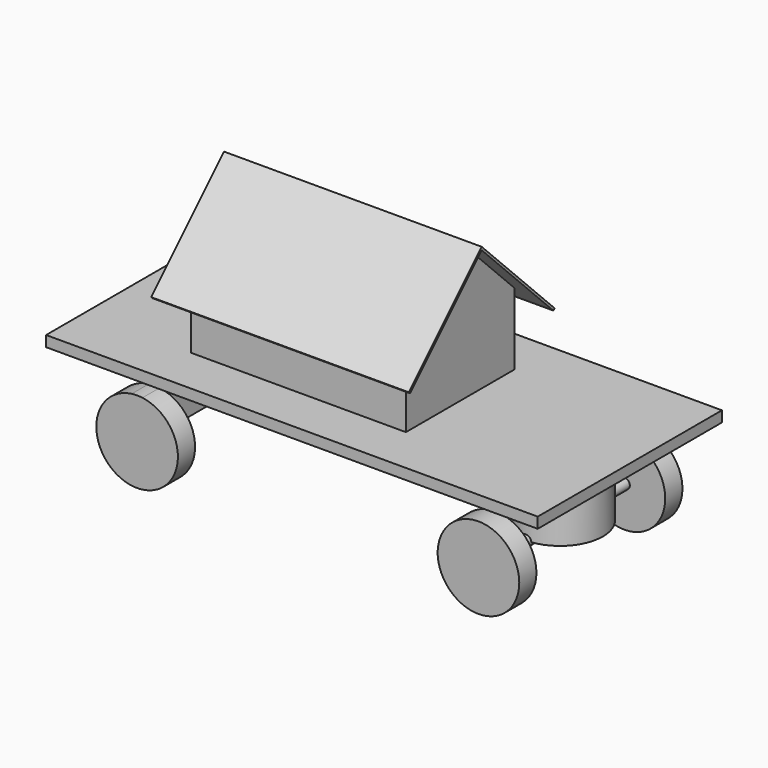
from build123d import *

# Parameters (mm, degrees)
F0_W      = 4580
F0_H      = 2145
F1_DEPTH  = 100
F2_W      = 100
F2_H      = 580
F3_DEPTH  = 450
F4_DEPTH  = 750
F6_DEPTH  = 200
F8_DEPTH  = 200
F9_R      = 400
F10_DEPTH = 580
F11_R     = 50
F12_DEPTH = 750
F13_R     = 380
F13_R_2   = 50
F14_DEPTH = 200
F15_R     = 380
F15_R_2   = 50
F16_DEPTH = 200
F17_W     = 2000
F17_H     = 1265
F18_DEPTH = 2000
F20_DEPTH = 2000
F22_DEPTH = 2200
F23_DEPTH = 200


# Not quite as in the source:
# - a feature names something its author has since deleted; it is built from what else it names


with BuildPart() as f1:
    # F0 (on Top) → F1 (new body)
    with BuildSketch(Plane.XY):
        Rectangle(F0_W, F0_H)
    extrude(amount=F1_DEPTH)

    # F2 (on Front) → F3 (join, symmetric)
    with BuildSketch(Plane.XZ):
        with Locations((-1540, -290)):
            Rectangle(F2_W, F2_H)
    extrude(amount=F3_DEPTH, both=True)

    # F2 (on Front) → F4 (join, symmetric)
    with BuildSketch(Plane.XZ):
        with Locations((-1540, -290)):
            Rectangle(F2_W, F2_H)
    extrude(amount=F4_DEPTH, both=True)

    # F5 (on face) → F6 (join)
    with BuildSketch(Plane.XZ.offset(750)):
        with BuildLine():
            ThreePointArc((-1590, -204.43457899), (-1790.399680511, -866.9628615859), (-1160, -581.1307430267))
            ThreePointArc((-1160, -581.1307430267), (-1254.1678814409, -330.7310625158), (-1490, -204.43457899))
            Line((-1490, -204.43457899), (-1490, -580))
            Line((-1490, -580), (-1590, -580))
            Line((-1590, -580), (-1590, -204.43457899))
        make_face()
        with BuildLine():
            Line((-1490, -580), (-1490, -204.43457899))
            ThreePointArc((-1490, -204.43457899), (-1540, -201.1307430267), (-1590, -204.43457899))
            Line((-1590, -204.43457899), (-1590, -580))
            Line((-1590, -580), (-1490, -580))
        make_face()
    extrude(amount=F6_DEPTH)

    # F7 (on face) → F8 (join)
    with BuildSketch(Plane(origin=(0, 750, 0), x_dir=(-1, 0, 0), z_dir=(0, 1, 0))):
        with BuildLine():
            Line((1590, -580), (1590, -203.3038359633))
            ThreePointArc((1590, -203.3038359633), (1540, -200), (1490, -203.3038359633))
            Line((1490, -203.3038359633), (1490, -580))
            Line((1490, -580), (1590, -580))
        make_face()
        with BuildLine():
            ThreePointArc((1490, -203.3038359633), (1289.600319489, -865.8321185591), (1920, -580))
            ThreePointArc((1920, -580), (1825.8321185591, -329.600319489), (1590, -203.3038359633))
            Line((1590, -203.3038359633), (1590, -580))
            Line((1590, -580), (1490, -580))
            Line((1490, -580), (1490, -203.3038359633))
        make_face()
    extrude(amount=F8_DEPTH)

    # F9 (on face) → F10 (join)
    with BuildSketch(Plane(origin=(0, 0, 0), x_dir=(1, 0, 0), z_dir=(0, 0, -1))):
        with Locations((1640, 0)):
            Circle(F9_R)
    extrude(amount=F10_DEPTH)

    # F11 (on Front) → F12 (join, symmetric)
    with BuildSketch(Plane.XZ):
        with Locations((1640, -580)):
            Circle(F11_R)
    extrude(amount=F12_DEPTH, both=True)

    # F13 (on face) → F14 (join)
    with BuildSketch(Plane.XZ.offset(750)):
        with Locations((1640, -580)):
            Circle(F13_R)
        with Locations((1640, -580)):
            Circle(F13_R_2, mode=Mode.SUBTRACT)
        with Locations((1640, -580)):
            Circle(F13_R_2)
    extrude(amount=F14_DEPTH)

    # F15 (on face) → F16 (join)
    with BuildSketch(Plane(origin=(0, 750, 0), x_dir=(-1, 0, 0), z_dir=(0, 1, 0))):
        with Locations((-1640, -580)):
            Circle(F15_R)
        with Locations((-1640, -580)):
            Circle(F15_R_2, mode=Mode.SUBTRACT)
        with Locations((-1640, -580)):
            Circle(F15_R_2)
    extrude(amount=F16_DEPTH)

    # F17 (on face) → F18 (join)
    with BuildSketch(Plane.XY.offset(100)):
        with Locations((-290, 0)):
            Rectangle(F17_W, F17_H)
    extrude(amount=F18_DEPTH)

    # F19 (on face) → F20 (cut)
    with BuildSketch(Plane.YZ.offset(710)):
        Polygon((-824.2233241082, 575.7766758918), (-632.5, 767.5), (-632.5, 2100), (632.5, 2100), (632.5, 767.5), (998.3408662269, 401.6591337731), (998.3408662269, 2239.1670500755), (-824.2233241082, 2239.1670500755), align=None)
        Polygon((-632.5, 767.5), (0, 1400), (632.5, 767.5), (632.5, 2100), (-632.5, 2100), align=None)
    extrude(amount=-F20_DEPTH, mode=Mode.SUBTRACT)

    # F21 (on face) → F22 (join)
    with BuildSketch(Plane.YZ.offset(710)):
        Polygon((-632.5, 767.5), (0, 1400), (632.5, 767.5), (834.3860018001, 565.6139981999), (848.5281374239, 579.7561338236), (0, 1428.2842712475), (-848.5281374239, 579.7561338236), (-834.3860018001, 565.6139981999), align=None)
    extrude(amount=-F22_DEPTH)

    # F21 (on face) → F23 (join)
    with BuildSketch(Plane.YZ.offset(710)):
        Polygon((-834.3860018001, 565.6139981999), (0, 1400), (834.3860018001, 565.6139981999), (848.5281374239, 579.7561338236), (0, 1428.2842712475), (-848.5281374239, 579.7561338236), align=None)
    extrude(amount=F23_DEPTH)


solid = f1.part
